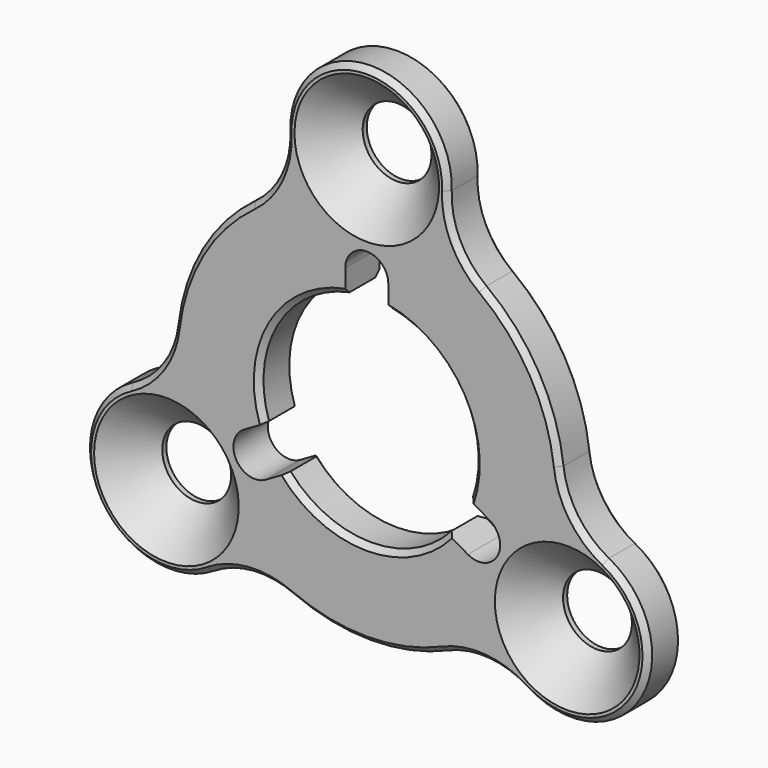
from build123d import *

# Parameters (mm, degrees)
F0_R           = 10
F1_DEPTH       = 2
F1_DEPTH_BACK  = 2
F2_SIZE        = 0.5
F4_D           = 6.4
F4_CSINK_D     = 13.44
F4_CSINK_ANGLE = 90
F6_DEPTH       = 4.001


# Not quite as in the source:
# - a feature names something its author has since deleted; it is built from what else it names


with BuildPart() as f1:
    # F0 (on Front) → F1 (new body, two sides)
    with BuildSketch(Plane.XZ) as f1_sk:
        with BuildLine():
            ThreePointArc((10.7222839925, 14.457960644), (8.271877925, 17.429551948), (7.4940694571, 21.2018004501))
            ThreePointArc((7.4940694571, 21.2018004501), (0, 29), (-7.4940694571, 21.2018004501))
            ThreePointArc((-7.4940694571, 21.2018004501), (-8.271877925, 17.429551948), (-10.7222839925, 14.457960644))
            ThreePointArc((-10.7222839925, 14.457960644), (-15.5884572681, 9), (-17.8821032009, 2.0567900021))
            ThreePointArc((-17.8821032009, 2.0567900021), (-19.2303737261, -1.551119554), (-22.1083325243, -4.1108456974))
            ThreePointArc((-22.1083325243, -4.1108456974), (-25.1147367097, -14.5), (-14.6142630672, -17.0909547527))
            ThreePointArc((-14.6142630672, -17.0909547527), (-10.9584958011, -15.8784323941), (-7.1598192084, -16.5147506461))
            ThreePointArc((-7.1598192084, -16.5147506461), (0, -18), (7.1598192084, -16.5147506461))
            ThreePointArc((7.1598192084, -16.5147506461), (10.9584958011, -15.8784323941), (14.6142630672, -17.0909547527))
            ThreePointArc((14.6142630672, -17.0909547527), (25.1147367097, -14.5), (22.1083325243, -4.1108456974))
            ThreePointArc((22.1083325243, -4.1108456974), (19.2303737261, -1.551119554), (17.8821032009, 2.0567900021))
            ThreePointArc((17.8821032009, 2.0567900021), (15.5884572681, 9), (10.7222839925, 14.457960644))
        make_face()
        Circle(F0_R, mode=Mode.SUBTRACT)
    extrude(amount=F1_DEPTH)
    extrude(f1_sk.sketch, amount=-F1_DEPTH_BACK)

    # F2
    f2_edges = [f1.edges().sort_by_distance(p)[0] for p in [
        (0, -2, 29),
        (0, 2, 29),
        (-10, -2, 0),
        (-10, 2, 0),
    ]]
    chamfer(f2_edges, length=F2_SIZE)

    # F4 (through all)
    with Locations(Plane.XZ.offset(2)):
        with Locations((0, 21.5), (-18.6195461814, -10.75), (18.6195461814, -10.75)):
            CounterSinkHole(F4_D / 2, F4_CSINK_D / 2, counter_sink_angle=F4_CSINK_ANGLE)

    # F5 (on face) → F6 (cut, through all)
    with BuildSketch(Plane.XZ.offset(2)):
        with BuildLine():
            ThreePointArc((-2, 9.7979589711), (0, 10), (2, 9.7979589711))
            Line((2, 9.7979589711), (2, 12))
            ThreePointArc((2, 12), (0, 14), (-2, 12))
            Line((-2, 12), (-2, 9.7979589711))
        make_face()
        with BuildLine():
            Line((-9.3923048454, -7.7320508076), (-7.4852813742, -6.6310302931))
            ThreePointArc((-7.4852813742, -6.6310302931), (-8.6602540378, -5), (-9.4852813742, -3.166928678))
            Line((-9.4852813742, -3.166928678), (-11.3923048454, -4.2679491924))
            ThreePointArc((-11.3923048454, -4.2679491924), (-12.124355653, -7), (-9.3923048454, -7.7320508076))
        make_face()
        with BuildLine():
            Line((11.3923048454, -4.2679491924), (9.4852813742, -3.166928678))
            ThreePointArc((9.4852813742, -3.166928678), (8.6602540378, -5), (7.4852813742, -6.6310302931))
            Line((7.4852813742, -6.6310302931), (9.3923048454, -7.7320508076))
            ThreePointArc((9.3923048454, -7.7320508076), (12.124355653, -7), (11.3923048454, -4.2679491924))
        make_face()
    extrude(amount=-F6_DEPTH, mode=Mode.SUBTRACT)


solid = f1.part
